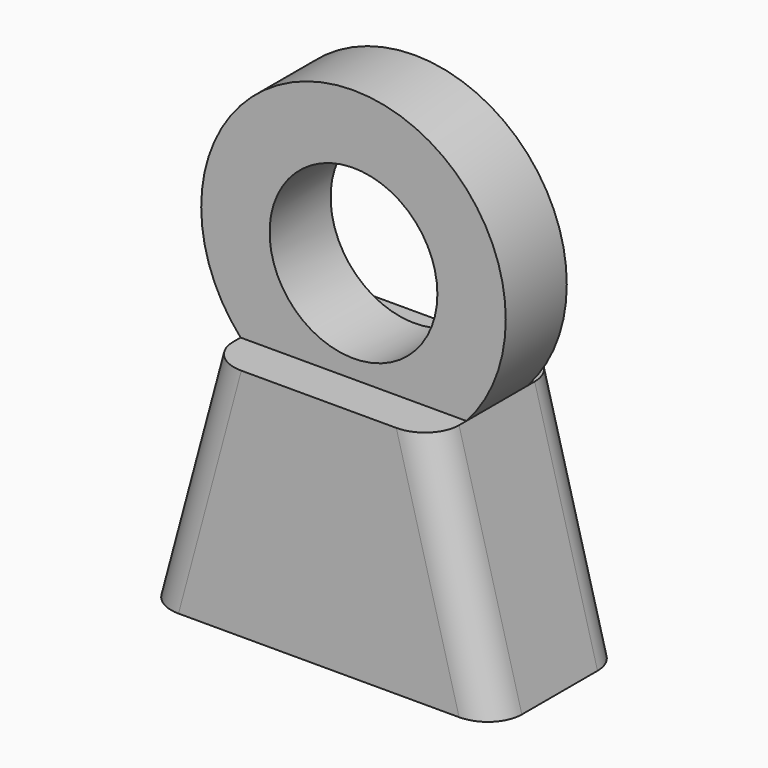
from build123d import *

# Parameters (mm, degrees)
F0_R     = 8.485
F0_R_2   = 4.675
F1_DEPTH = 2.125
F3_DEPTH = 4.539996
F5_DEPTH = 2.0625
F6_R     = 2.06249
F7_R     = 1.905


# Not quite as in the source:
# - a fillet or chamfer is up to 0.001 mm smaller than in the source, because OpenCascade refuses the exact size


with BuildPart() as f1:
    # F0 (on Front) → F1 (new body, symmetric)
    with BuildSketch(Plane.XZ):
        Circle(F0_R)
        Circle(F0_R_2, mode=Mode.SUBTRACT)
    extrude(amount=F1_DEPTH, both=True)

    # F2 (on Front) → F3 (join, symmetric)
    with BuildSketch(Plane.XZ):
        Polygon((-6.2906053879, -5.6941644561), (-9.7885362858, -18.7486202883), (9.7885362858, -18.7486202883), (6.2906053879, -5.6941644561), align=None)
    extrude(amount=F3_DEPTH, both=True)

    # F4 (on Front) → F5 (cut, symmetric)
    with BuildSketch(Plane.XZ):
        Polygon((4.22592549, -7.8024805709), (0.2414814566, -8.8701091319), (2.8884205433, -18.7486202883), (7.1589347875, -18.7486202883), align=None)
        Polygon((-0.2414814566, -8.8701091319), (-4.22592549, -7.8024805709), (-6.8555269883, -17.6162869659), (-7.1589347875, -18.7486202883), (-2.8884205433, -18.7486202883), align=None)
    extrude(amount=F5_DEPTH, both=True, mode=Mode.SUBTRACT)

    # F6 (radius 2.0625 in the source; OpenCascade refuses exactly that, so slightly less here)
    f6_edges = [f1.edges().sort_by_distance(p)[0] for p in [
        (-5.69243, -2.0625, -13.27555),
        (1.564951, -2.0625, -13.809365),
        (5.69243, -2.0625, -13.27555),
        (-1.564951, -2.0625, -13.809365),
        (5.69243, 2.0625, -13.27555),
        (-1.564951, 2.0625, -13.809365),
        (-5.69243, 2.0625, -13.27555),
        (1.564951, 2.0625, -13.809365),
    ]]
    fillet(f6_edges, radius=F6_R)

    # F7
    f7_edges = [f1.edges().sort_by_distance(p)[0] for p in [
        (8.039571, 4.539996, -12.221392),
        (8.039571, -4.539996, -12.221392),
        (-8.039571, 4.539996, -12.221392),
        (-8.039571, -4.539996, -12.221392),
    ]]
    fillet(f7_edges, radius=F7_R)


solid = f1.part
